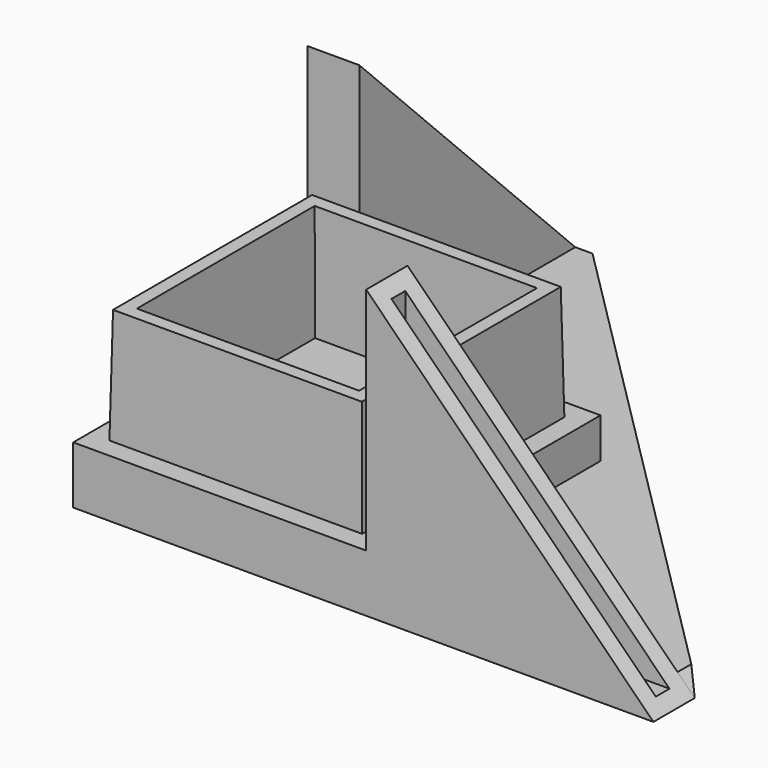
from build123d import *

# Parameters (mm, degrees)
F0_W      = 51
F0_H      = 51
F1_DEPTH  = 10
F4_DEPTH  = 4.5
F6_DEPTH  = 1.5
F9_DEPTH  = 4.5
F11_DEPTH = 1.5
F12_W     = 44
F12_H     = 44
F12_W_2   = 38
F12_H_2   = 38
F13_DEPTH = 20
F13_TAPER = 1
F15_DEPTH = 3
F17_DEPTH = 25
F19_DEPTH = 25


with BuildPart() as f1:
    # F0 (on Top) → F1 (new body)
    with BuildSketch(Plane.XY):
        Rectangle(F0_W, F0_H)
    extrude(amount=F1_DEPTH)

    # F3 (on offset) → F4 (join, symmetric)
    with BuildSketch(Plane.XZ.offset(21)):
        Polygon((25.5, 50), (25.5, 0), (75.5, 0), align=None)
    extrude(amount=F4_DEPTH, both=True)

    # F5 (on offset) → F6 (cut, symmetric)
    with BuildSketch(Plane.XZ.offset(21)):
        Polygon((73.5, 2), (27.5, 48), (27.5, 2), align=None)
    extrude(amount=F6_DEPTH, both=True, mode=Mode.SUBTRACT)

    # F8 (on offset) → F9 (join, symmetric)
    with BuildSketch(Plane.YZ.offset(-21)):
        Polygon((25.5, 50), (25.5, 0), (75.5, 0), align=None)
    extrude(amount=F9_DEPTH, both=True)

    # F10 (on offset) → F11 (cut, symmetric)
    with BuildSketch(Plane.YZ.offset(-21)):
        Polygon((27.5, 48), (27.5, 2), (73.5, 2), align=None)
    extrude(amount=F11_DEPTH, both=True, mode=Mode.SUBTRACT)

    # F12 (on face) → F13 (join)
    with BuildSketch(Plane.XY.offset(10)):
        Rectangle(F12_W, F12_H)
        Rectangle(F12_W_2, F12_H_2, mode=Mode.SUBTRACT)
    extrude(amount=F13_DEPTH, taper=F13_TAPER)


with BuildPart() as f15:
    # F14 (on face) → F15 (new body)
    with BuildSketch(Plane(origin=(0, 0, 0), x_dir=(1, 0, 0), z_dir=(0, 0, -1))):
        Polygon((-16.5, -25.5), (-16.5, -75.5), (75.5, 16.5), (25.5, 16.5), (25.5, -25.5), align=None)
    extrude(amount=-F15_DEPTH)

    # F16 (on face) → F17 (cut)
    with BuildSketch(Plane(origin=(-16.5, 0, 0), x_dir=(0, -1, 0), z_dir=(-1, 0, 0))):
        Polygon((-72.5, 3), (-75.5, 3), (-75.5, 0), align=None)
    extrude(amount=-F17_DEPTH, mode=Mode.SUBTRACT)

    # F18 (on face) → F19 (cut)
    with BuildSketch(Plane.XZ.offset(16.5)):
        Polygon((75.5, 0), (75.5, 3), (72.5, 3), align=None)
    extrude(amount=-F19_DEPTH, mode=Mode.SUBTRACT)


solid = Compound([f1.part, f15.part])
